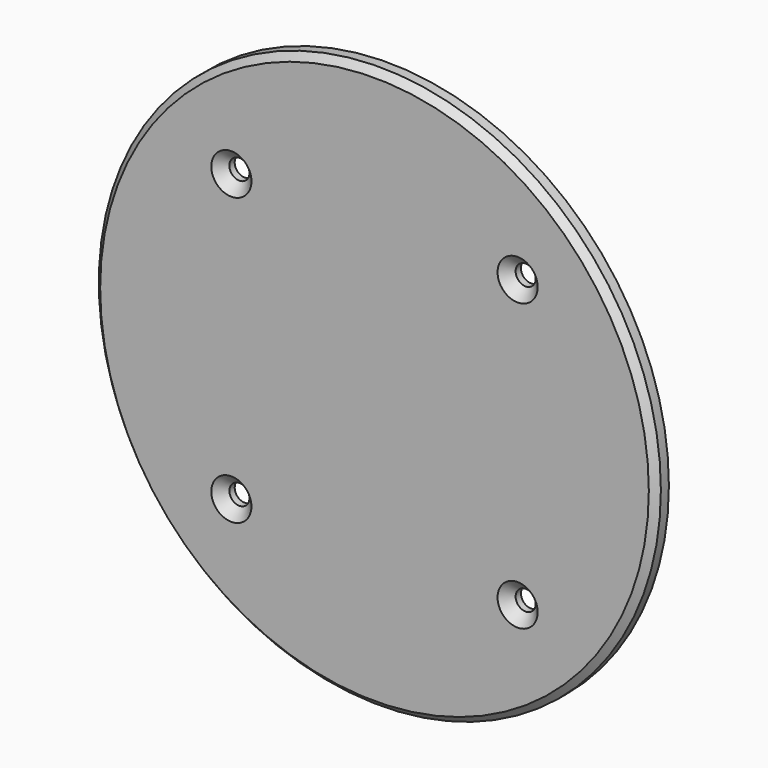
from build123d import *

# Parameters (mm, degrees)
F0_R     = 84
F0_R_2   = 3
F1_DEPTH = 5
F2_SIZE  = 2
F3_SIZE  = 3


# Not quite as in the source:
# - a feature names something its author has since deleted; it is built from what else it names


with BuildPart() as f1:
    # F0 (on Front) → F1 (new body)
    with BuildSketch(Plane.XZ):
        Circle(F0_R)
        with Locations((-42.7799602618, -42.7799602618)):
            Circle(F0_R_2, mode=Mode.SUBTRACT)
        with Locations((42.7799602618, -42.7799602618)):
            Circle(F0_R_2, mode=Mode.SUBTRACT)
        with Locations((-42.7799602618, 42.7799602618)):
            Circle(F0_R_2, mode=Mode.SUBTRACT)
        with Locations((42.7799602618, 42.7799602618)):
            Circle(F0_R_2, mode=Mode.SUBTRACT)
    extrude(amount=F1_DEPTH)

    # F2
    f2_edges = [f1.edges().sort_by_distance(p)[0] for p in [
        (-84, -5, 0),
    ]]
    chamfer(f2_edges, length=F2_SIZE)

    # F3
    f3_edges = [f1.edges().sort_by_distance(p)[0] for p in [
        (-45.77996, -5, 42.77996),
        (39.77996, -5, 42.77996),
        (-45.77996, -5, -42.77996),
        (39.77996, -5, -42.77996),
    ]]
    chamfer(f3_edges, length=F3_SIZE)


solid = f1.part
